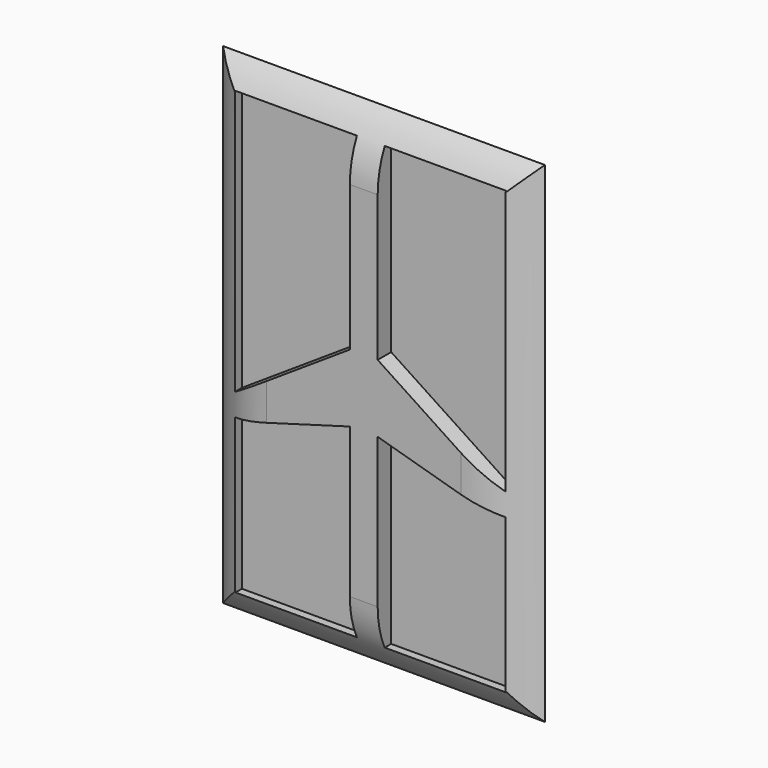
from build123d import *

# Parameters (mm, degrees)
F1_DEPTH    = 6
F0_W        = 76.4068576
F0_H        = 116.405787
F2_DEPTH    = 6
F3_DEPTH    = 2
F4_T1_DEPTH = 192.098587186
F4_T3_DEPTH = 152.099657786


# Not quite as in the source:
# - a fillet or chamfer that OpenCascade refuses, or shapes differently, is made with other operations: its cross-section is extruded or revolved along the edge and cut away or added
# - a feature names something its author has since deleted; it is built from what else it names


with BuildPart() as f1:
    # F0 (on Front) → F1 (new body)
    with BuildSketch(Plane.XZ):
        Polygon((15.6125306649, 37.6914590597), (9.0085306649, 37.6914590597), (9.0085306649, -6.1789248552), (-19.818228389, -25.1597724855), (-19.818228389, -30.4937724855), (9.0085306649, -22.2596581395), (9.0085306649, -67.1633433111), (15.6125306649, -67.1633433111), (15.6125306649, -22.2596581395), (44.4392897189, -30.4937724855), (44.4392897189, -25.1597724855), (15.6125306649, -6.1789248552), align=None)
    extrude(amount=F1_DEPTH)

    # F0 (on Front) → F2 (join)
    with BuildSketch(Plane.XZ):
        with Locations((12.3105306649, -14.7359421257)):
            Rectangle(F0_W, F0_H)
        Polygon((-19.818228389, -25.1597724855), (-19.818228389, 37.6914590597), (9.0085306649, 37.6914590597), (15.6125306649, 37.6914590597), (44.4392897189, 37.6914590597), (44.4392897189, -25.1597724855), (44.4392897189, -30.4937724855), (44.4392897189, -67.1633433111), (15.6125306649, -67.1633433111), (9.0085306649, -67.1633433111), (-19.818228389, -67.1633433111), (-19.818228389, -30.4937724855), align=None, mode=Mode.SUBTRACT)
    extrude(amount=F2_DEPTH)

    # F0 (on Front) → F3 (join)
    with BuildSketch(Plane.XZ):
        Polygon((9.0085306649, 37.6914590597), (-19.818228389, 37.6914590597), (-19.818228389, -25.1597724855), (9.0085306649, -6.1789248552), align=None)
        Polygon((44.4392897189, -67.1633433111), (44.4392897189, -30.4937724855), (15.6125306649, -22.2596581395), (15.6125306649, -67.1633433111), align=None)
        Polygon((9.0085306649, -22.2596581395), (-19.818228389, -30.4937724855), (-19.818228389, -67.1633433111), (9.0085306649, -67.1633433111), align=None)
        Polygon((44.4392897189, 37.6914590597), (15.6125306649, 37.6914590597), (15.6125306649, -6.1789248552), (44.4392897189, -25.1597724855), align=None)
    extrude(amount=F3_DEPTH)

    # F4: fillet of radius 22.098 on 4 edges, made by hand

    # F4_s2 → F4_t1 (cut)
    with BuildSketch(Plane.XY.offset(-110.7852357187)):
        with BuildLine():
            ThreePointArc((-25.8928981351, 0), (-18.8964508458, -4.445310444), (-10.7543380979, -6))
            Line((-10.7543380979, -6), (-25.8928981351, -6))
            Line((-25.8928981351, -6), (-25.8928981351, 0))
        make_face()
        with BuildLine():
            ThreePointArc((50.5139594649, 0), (43.5175121757, -4.445310444), (35.3753994277, -6))
            Line((35.3753994277, -6), (50.5139594649, -6))
            Line((50.5139594649, -6), (50.5139594649, 0))
        make_face()
    extrude(amount=F4_T1_DEPTH, mode=Mode.SUBTRACT)

    # F4_s4 → F4_t3 (cut)
    with BuildSketch(Plane.YZ.offset(-63.7392982281)):
        with BuildLine():
            ThreePointArc((0, -72.9388356257), (-4.445310444, -65.9423883364), (-6, -57.8002755885))
            Line((-6, -57.8002755885), (-6, -72.9388356257))
            Line((-6, -72.9388356257), (0, -72.9388356257))
        make_face()
        with BuildLine():
            ThreePointArc((-6, 28.3283913371), (-4.445310444, 36.4705040851), (0, 43.4669513743))
            Line((0, 43.4669513743), (-6, 43.4669513743))
            Line((-6, 43.4669513743), (-6, 28.3283913371))
        make_face()
    extrude(amount=F4_T3_DEPTH, mode=Mode.SUBTRACT)


solid = f1.part
